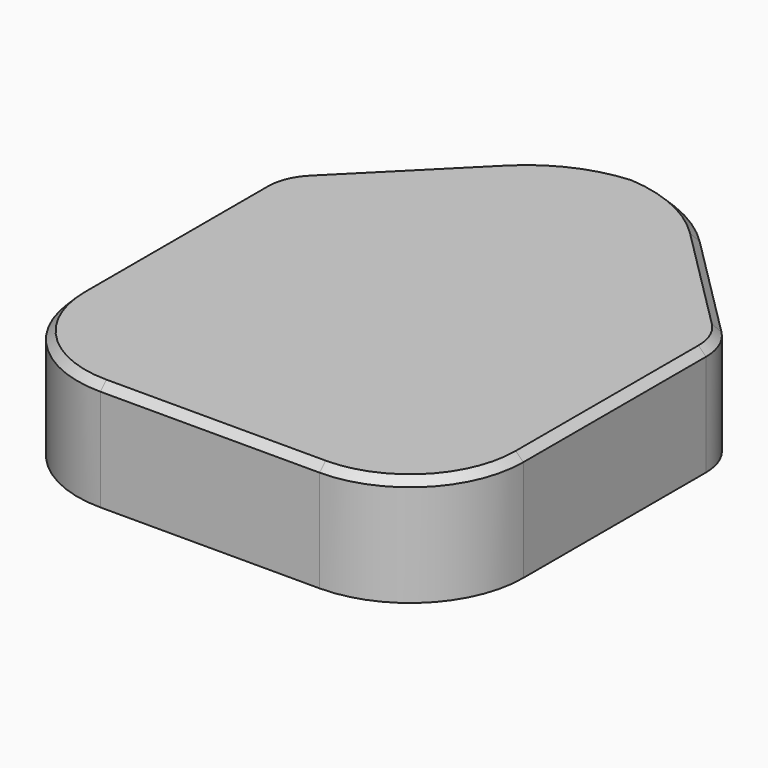
from build123d import *

# Parameters (mm, degrees)
F0_W         = 150
F0_H         = 180.0098
F1_DEPTH     = 36.83
F2_R         = 38.1
F3_R         = 38.1
F4_SIZE      = 57.15
F5_SIZE      = 57.15
F6_T         = -4.826
F7_T1_DEPTH  = 142.0402448428
F8_R         = 19.05
F9_T1_DEPTH  = 51.8894877579
F9_T3_DEPTH  = 76.8690316368
F9_T5_DEPTH  = 73.8
F9_T7_DEPTH  = 51.8894877579
F9_T10_ANGLE = 78.2371868637
F9_T12_ANGLE = 78.2371868637
F9_T14_ANGLE = 45
F9_T16_ANGLE = 90
F9_T18_ANGLE = 90
F9_T20_ANGLE = 45


# Not quite as in the source:
# - a fillet or chamfer that OpenCascade refuses, or shapes differently, is made with other operations: its cross-section is extruded or revolved along the edge and cut away or added


with BuildPart() as f1:
    # F0 (on Top) → F1 (new body)
    with BuildSketch(Plane.XY):
        with Locations((-75, 90.0049)):
            Rectangle(F0_W, F0_H)
    extrude(amount=F1_DEPTH)

    # F2
    f2_edges = [f1.edges().sort_by_distance(p)[0] for p in [
        (0, 0, 18.415),
    ]]
    fillet(f2_edges, radius=F2_R)

    # F3
    f3_edges = [f1.edges().sort_by_distance(p)[0] for p in [
        (-150, 0, 18.415),
    ]]
    fillet(f3_edges, radius=F3_R)

    # F4
    f4_edges = [f1.edges().sort_by_distance(p)[0] for p in [
        (-150, 180.0098, 18.415),
    ]]
    chamfer(f4_edges, length=F4_SIZE)

    # F5
    f5_edges = [f1.edges().sort_by_distance(p)[0] for p in [
        (0, 180.0098, 18.415),
    ]]
    chamfer(f5_edges, length=F5_SIZE)

    # F6
    f6_openings = [f1.faces().sort_by_distance(p)[0] for p in [
        (-75, 82.174731, 0),
    ]]
    offset(amount=F6_T, openings=f6_openings)

    # F7: fillet of radius 50.8 on 2 edges, made by hand

    # F7_s2 → F7_t1 (cut)
    with BuildSketch(Plane.XY.offset(-52.6051224214)):
        with BuildLine():
            ThreePointArc((-71.8079510314, 180.0098), (-91.2482693956, 176.1428802516), (-107.7289755157, 165.1308244843))
            Line((-107.7289755157, 165.1308244843), (-92.85, 180.0098))
            Line((-92.85, 180.0098), (-71.8079510314, 180.0098))
        make_face()
        with BuildLine():
            ThreePointArc((-78.1920489686, 180.0098), (-58.7517306044, 176.1428802516), (-42.2710244843, 165.1308244843))
            Line((-42.2710244843, 165.1308244843), (-57.15, 180.0098))
            Line((-57.15, 180.0098), (-78.1920489686, 180.0098))
        make_face()
    extrude(amount=F7_T1_DEPTH, mode=Mode.SUBTRACT)

    # F8
    f8_edges = [f1.edges().sort_by_distance(p)[0] for p in [
        (-150, 122.8598, 18.415),
        (0, 122.8598, 18.415),
    ]]
    fillet(f8_edges, radius=F8_R)

    # F9: chamfer of 2.54 on 10 edges, made by hand

    # F9_s2 → F9_t1 (cut)
    with BuildSketch(Plane(origin=(-7.9904841816, -7.9904841816, 0), x_dir=(0, 0, 1), z_dir=(0.7071067812, 0.7071067812, 0))):
        Polygon((34.29, -192.9410148932), (36.83, -190.4010148932), (36.83, -192.9410148932), align=None)
    extrude(amount=F9_T1_DEPTH, mode=Mode.SUBTRACT)

    # F9_s4 → F9_t3 (cut)
    with BuildSketch(Plane.XZ.offset(-114.9690316368)):
        Polygon((-150, 34.29), (-147.46, 36.83), (-150, 36.83), align=None)
        Polygon((0, 34.29), (-2.54, 36.83), (0, 36.83), align=None)
    extrude(amount=F9_T3_DEPTH, mode=Mode.SUBTRACT)

    # F9_s6 → F9_t5 (cut)
    with BuildSketch(Plane.YZ.offset(-111.9)):
        Polygon((0, 34.29), (2.54, 36.83), (0, 36.83), align=None)
    extrude(amount=F9_T5_DEPTH, mode=Mode.SUBTRACT)

    # F9_s8 → F9_t7 (cut)
    with BuildSketch(Plane(origin=(-103.7009244843, 103.7009244843, 0), x_dir=(0, 0, 1), z_dir=(0.7071067812, -0.7071067812, 0))):
        Polygon((34.29, -86.8749977152), (36.83, -84.3349977152), (36.83, -86.8749977152), align=None)
    extrude(amount=F9_T7_DEPTH, mode=Mode.SUBTRACT)

    # F9_s9 → F9_t10 (revolve, cut)
    with BuildSketch(Plane(origin=(4.5334842912, 2.9708331336, 0), x_dir=(0, 0, 1), z_dir=(-0.8364087505, -0.548106196, 0))):
        Polygon((34.29, 201.7297538876), (36.83, 199.1897538876), (36.83, 201.7297538876), align=None)
    revolve(axis=Axis((-78.1920489684, 129.2098000003, 36.83), (0, 0, -1)), revolution_arc=F9_T10_ANGLE, mode=Mode.SUBTRACT)

    # F9_s11 → F9_t12 (revolve, cut)
    with BuildSketch(Plane(origin=(28.7009244845, 28.7009244846, 0), x_dir=(0, 0, 1), z_dir=(-0.7071067812, -0.7071067812, 0))):
        Polygon((34.29, 192.9410148931), (36.83, 190.4010148931), (36.83, 192.9410148931), align=None)
    revolve(axis=Axis((-71.8079510316, 129.2098000003, 36.83), (0, 0, -1)), revolution_arc=F9_T12_ANGLE, mode=Mode.SUBTRACT)

    # F9_s13 → F9_t14 (revolve, cut)
    with BuildSketch(Plane.XZ.offset(-114.9690316368)):
        Polygon((-150, 34.29), (-147.46, 36.83), (-150, 36.83), align=None)
    revolve(axis=Axis((-130.95, 114.9690316368, 36.83), (0, 0, -1)), revolution_arc=F9_T14_ANGLE, mode=Mode.SUBTRACT)

    # F9_s15 → F9_t16 (revolve, cut)
    with BuildSketch(Plane.YZ.offset(-111.9)):
        Polygon((0, 34.29), (2.54, 36.83), (0, 36.83), align=None)
    revolve(axis=Axis((-111.9, 38.1, 36.83), (0, 0, -1)), revolution_arc=F9_T16_ANGLE, mode=Mode.SUBTRACT)

    # F9_s17 → F9_t18 (revolve, cut)
    with BuildSketch(Plane.YZ.offset(-38.1)):
        Polygon((0, 34.29), (2.54, 36.83), (0, 36.83), align=None)
    revolve(axis=Axis((-38.1, 38.1, 36.83), (0, 0, 1)), revolution_arc=F9_T18_ANGLE, mode=Mode.SUBTRACT)

    # F9_s19 → F9_t20 (revolve, cut)
    with BuildSketch(Plane(origin=(-67.0095158184, 67.0095158184, 0), x_dir=(0, 0, 1), z_dir=(-0.7071067812, 0.7071067812, 0))):
        Polygon((34.29, 86.8749977152), (36.83, 84.3349977152), (36.83, 86.8749977152), align=None)
    revolve(axis=Axis((-19.05, 114.9690316368, 36.83), (0, 0, -1)), revolution_arc=F9_T20_ANGLE, mode=Mode.SUBTRACT)


solid = f1.part
